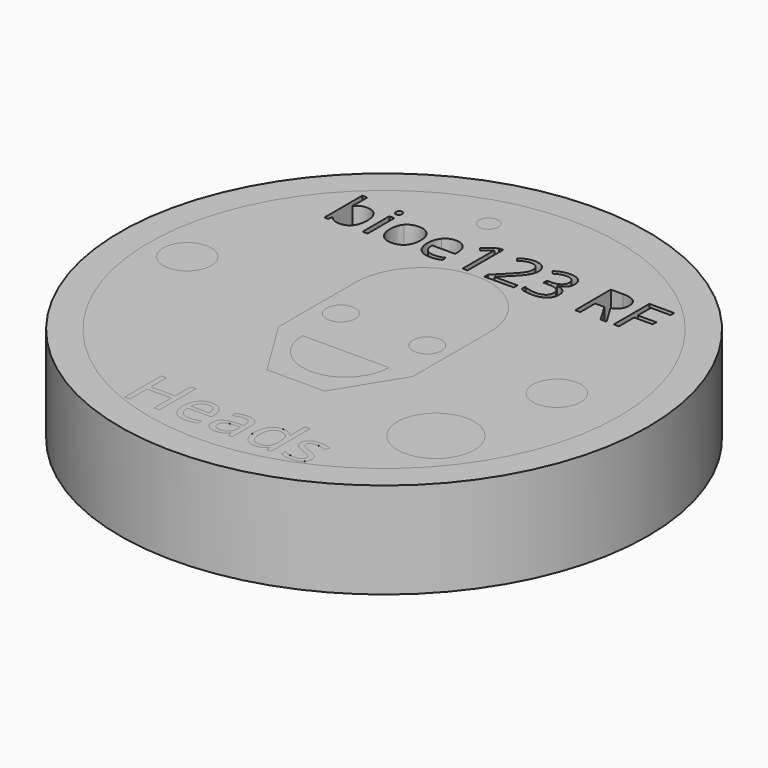
from build123d import *

# Parameters (mm, degrees)
F0_R         = 27.5
F0_R_2       = 24.5
F0_TEXT_SIZE = 6.6889777583
F0_R_3       = 4
F0_R_4       = 2.5
F0_R_5       = 1.5
F0_R_6       = 1
F1_DEPTH     = 10
F0_W         = 0.5273596823
F0_H         = 3.48016746
F2_DEPTH     = 2
F3_DEPTH     = 8


# Not quite as in the source:
# - Text() gives the source's letters only with a copy of the font that has no kerning and outlines rounded to 1/6400 em; it was checked with that copy


with BuildPart() as f1:
    # F0 (on Top) → F1 (new body)
    with BuildSketch(Plane.XY):
        Circle(F0_R)
        Circle(F0_R_2, mode=Mode.SUBTRACT)
        with Locations((-9.6953597148, -22.5)):
            Text('Heads', F0_TEXT_SIZE, font='Open Sans', text_align=(TextAlign.LEFT, TextAlign.BOTTOM))
        with Locations((15, -12)):
            Circle(F0_R_3)
        with Locations((18, 0)):
            Circle(F0_R_4)
        with BuildLine():
            Line((-3, -11.5), (3, -11.5))
            Line((3, -11.5), (7, -5))
            Line((7, -5), (7, 5))
            ThreePointArc((7, 5), (0, 12), (-7, 5))
            Line((-7, 5), (-7, -5))
            Line((-7, -5), (-3, -11.5))
        make_face()
        with BuildLine():
            Line((-4.5, -5), (4.5, -5))
            ThreePointArc((4.5, -5), (0, -9.5), (-4.5, -5))
        make_face(mode=Mode.SUBTRACT)
        with Locations((-4.5, 0)):
            Circle(F0_R_5, mode=Mode.SUBTRACT)
        with Locations((4.5, 0)):
            Circle(F0_R_5, mode=Mode.SUBTRACT)
        with Locations((-20.5, 0)):
            Circle(F0_R_4)
        with Locations((-5, 19.8808953521)):
            Circle(F0_R_6)
    extrude(amount=F1_DEPTH)

    # F0 (on Top) → F2 (join)
    with BuildSketch(Plane.XY):
        Circle(F0_R_2)
        with BuildLine():
            add(Edge.make_bspline(
                [(-2.0542477787, -22.5114966805), (-2.3103102086, -22.5658446248), (-2.6729782214, -22.5658446248)],
                knots=[0, 0, 0, 1, 1, 1], degree=2))
            add(Edge.make_bspline(
                [(-2.6729782214, -22.5658446248), (-3.4662491774, -22.5658446248), (-3.9255938219, -22.0819388901)],
                knots=[0, 0, 0, 1, 1, 1], degree=2))
            add(Edge.make_bspline(
                [(-3.9255938219, -22.0819388901), (-4.3849384664, -21.5980331554), (-4.3849384664, -20.7399627273)],
                knots=[0, 0, 0, 1, 1, 1], degree=2))
            add(Edge.make_bspline(
                [(-4.3849384664, -20.7399627273), (-4.3849384664, -19.8735310771), (-3.9585161343, -19.3640190994)],
                knots=[0, 0, 0, 1, 1, 1], degree=2))
            add(Edge.make_bspline(
                [(-3.9585161343, -19.3640190994), (-3.5320938022, -18.8545071217), (-2.8130286932, -18.8545071217)],
                knots=[0, 0, 0, 1, 1, 1], degree=2))
            add(Edge.make_bspline(
                [(-2.8130286932, -18.8545071217), (-2.140995459, -18.8545071217), (-1.7490631685, -19.2971293218)],
                knots=[0, 0, 0, 1, 1, 1], degree=2))
            add(Edge.make_bspline(
                [(-1.7490631685, -19.2971293218), (-1.357130878, -19.7397515219), (-1.357130878, -20.4650875476)],
                knots=[0, 0, 0, 1, 1, 1], degree=2))
            Line((-1.357130878, -20.4650875476), (-1.357130878, -20.8078976577))
            Line((-1.357130878, -20.8078976577), (-3.8226462736, -20.8078976577))
            add(Edge.make_bspline(
                [(-3.8226462736, -20.8078976577), (-3.8059238292, -21.4381247809), (-3.5038746773, -21.764735023)],
                knots=[0, 0, 0, 1, 1, 1], degree=2))
            add(Edge.make_bspline(
                [(-3.5038746773, -21.764735023), (-3.2018255254, -22.0913452651), (-2.6531203187, -22.0913452651)],
                knots=[0, 0, 0, 1, 1, 1], degree=2))
            add(Edge.make_bspline(
                [(-2.6531203187, -22.0913452651), (-2.0751508342, -22.0913452651), (-1.5107683359, -21.8499149741)],
                knots=[0, 0, 0, 1, 1, 1], degree=2))
            Line((-1.5107683359, -21.8499149741), (-1.5107683359, -22.3338207088))
            add(Edge.make_bspline(
                [(-1.5107683359, -22.3338207088), (-1.7981853489, -22.4571487362), (-2.0542477787, -22.5114966805)],
                knots=[0, 0, 0, 1, 1, 1], degree=2))
        make_face(mode=Mode.SUBTRACT)
        Polygon((-5.4133687967, -17.7246969722), (-5.4133687967, -22.5), (-5.9683449201, -22.5), (-5.9683449201, -20.2529215343), (-8.4840276489, -20.2529215343), (-8.4840276489, -22.5), (-9.0390037723, -22.5), (-9.0390037723, -17.7246969722), (-8.4840276489, -17.7246969722), (-8.4840276489, -19.7564739663), (-5.9683449201, -19.7564739663), (-5.9683449201, -17.7246969722), align=None, mode=Mode.SUBTRACT)
        with BuildLine():
            Line((2.1713048895, -22.5), (1.7689210712, -22.5))
            Line((1.7689210712, -22.5), (1.6612703354, -21.9899654459))
            Line((1.6612703354, -21.9899654459), (1.6351415161, -21.9899654459))
            add(Edge.make_bspline(
                [(1.6351415161, -21.9899654459), (1.3675824057, -22.3265046394), (1.1015910246, -22.4461746321)],
                knots=[0, 0, 0, 1, 1, 1], degree=2))
            add(Edge.make_bspline(
                [(1.1015910246, -22.4461746321), (0.8355996434, -22.5658446248), (0.4363512835, -22.5658446248)],
                knots=[0, 0, 0, 1, 1, 1], degree=2))
            add(Edge.make_bspline(
                [(0.4363512835, -22.5658446248), (-0.0956314789, -22.5658446248), (-0.3976806308, -22.2909694451)],
                knots=[0, 0, 0, 1, 1, 1], degree=2))
            add(Edge.make_bspline(
                [(-0.3976806308, -22.2909694451), (-0.6997297827, -22.0160942653), (-0.6997297827, -21.5102403223)],
                knots=[0, 0, 0, 1, 1, 1], degree=2))
            add(Edge.make_bspline(
                [(-0.6997297827, -21.5102403223), (-0.6997297827, -20.4264168949), (1.0341786706, -20.3741592562)],
                knots=[0, 0, 0, 1, 1, 1], degree=2))
            Line((1.0341786706, -20.3741592562), (1.6414124327, -20.3543013535))
            Line((1.6414124327, -20.3543013535), (1.6414124327, -20.1316838124))
            add(Edge.make_bspline(
                [(1.6414124327, -20.1316838124), (1.6414124327, -19.7104872442), (1.4606010027, -19.5098179115)],
                knots=[0, 0, 0, 1, 1, 1], degree=2))
            add(Edge.make_bspline(
                [(1.4606010027, -19.5098179115), (1.2797895727, -19.3091485787), (0.8805412127, -19.3091485787)],
                knots=[0, 0, 0, 1, 1, 1], degree=2))
            add(Edge.make_bspline(
                [(0.8805412127, -19.3091485787), (0.4332158251, -19.3091485787), (-0.1311666732, -19.5829786057)],
                knots=[0, 0, 0, 1, 1, 1], degree=2))
            Line((-0.1311666732, -19.5829786057), (-0.2983911172, -19.1680529541))
            add(Edge.make_bspline(
                [(-0.2983911172, -19.1680529541), (-0.0339674652, -19.024867024), (0.2811460964, -18.9433451076)],
                knots=[0, 0, 0, 1, 1, 1], degree=2))
            add(Edge.make_bspline(
                [(0.2811460964, -18.9433451076), (0.596259658, -18.8618231911), (0.9139861015, -18.8618231911)],
                knots=[0, 0, 0, 1, 1, 1], degree=2))
            add(Edge.make_bspline(
                [(0.9139861015, -18.8618231911), (1.5536195996, -18.8618231911), (1.8624622446, -19.1455821695)],
                knots=[0, 0, 0, 1, 1, 1], degree=2))
            add(Edge.make_bspline(
                [(1.8624622446, -19.1455821695), (2.1713048895, -19.4293411478), (2.1713048895, -20.0564328127)],
                knots=[0, 0, 0, 1, 1, 1], degree=2))
            Line((2.1713048895, -20.0564328127), (2.1713048895, -22.5))
        make_face(mode=Mode.SUBTRACT)
        with BuildLine():
            add(Edge.make_bspline(
                [(9.471697021, -20.9322708379), (9.6953597148, -21.1674302122), (9.6953597148, -21.5238273084)],
                knots=[0, 0, 0, 1, 1, 1], degree=2))
            add(Edge.make_bspline(
                [(9.6953597148, -21.5238273084), (9.6953597148, -22.0234103347), (9.323285327, -22.2946274798)],
                knots=[0, 0, 0, 1, 1, 1], degree=2))
            add(Edge.make_bspline(
                [(9.323285327, -22.2946274798), (8.9512109392, -22.5658446248), (8.2781325523, -22.5658446248)],
                knots=[0, 0, 0, 1, 1, 1], degree=2))
            add(Edge.make_bspline(
                [(8.2781325523, -22.5658446248), (7.5663835127, -22.5658446248), (7.1681803055, -22.3400916255)],
                knots=[0, 0, 0, 1, 1, 1], degree=2))
            Line((7.1681803055, -22.3400916255), (7.1681803055, -21.8373731408))
            add(Edge.make_bspline(
                [(7.1681803055, -21.8373731408), (7.4263330409, -21.9680172377), (7.7215886997, -22.0427456611)],
                knots=[0, 0, 0, 1, 1, 1], degree=2))
            add(Edge.make_bspline(
                [(7.7215886997, -22.0427456611), (8.0168443586, -22.1174740844), (8.2917195384, -22.1174740844)],
                knots=[0, 0, 0, 1, 1, 1], degree=2))
            add(Edge.make_bspline(
                [(8.2917195384, -22.1174740844), (8.7160515649, -22.1174740844), (8.9444174462, -21.9821268001)],
                knots=[0, 0, 0, 1, 1, 1], degree=2))
            add(Edge.make_bspline(
                [(8.9444174462, -21.9821268001), (9.1727833275, -21.8467795158), (9.1727833275, -21.5687688777)],
                knots=[0, 0, 0, 1, 1, 1], degree=2))
            add(Edge.make_bspline(
                [(9.1727833275, -21.5687688777), (9.1727833275, -21.3597383228), (8.9919718974, -21.2113266288)],
                knots=[0, 0, 0, 1, 1, 1], degree=2))
            add(Edge.make_bspline(
                [(8.9919718974, -21.2113266288), (8.8111604674, -21.0629149347), (8.2844034689, -20.8601552964)],
                knots=[0, 0, 0, 1, 1, 1], degree=2))
            add(Edge.make_bspline(
                [(8.2844034689, -20.8601552964), (7.7848204426, -20.6741181025), (7.5742221585, -20.5351127835)],
                knots=[0, 0, 0, 1, 1, 1], degree=2))
            add(Edge.make_bspline(
                [(7.5742221585, -20.5351127835), (7.3636238744, -20.3961074645), (7.2606763261, -20.2199992219)],
                knots=[0, 0, 0, 1, 1, 1], degree=2))
            add(Edge.make_bspline(
                [(7.2606763261, -20.2199992219), (7.1577287778, -20.0438909794), (7.1577287778, -19.7993252301)],
                knots=[0, 0, 0, 1, 1, 1], degree=2))
            add(Edge.make_bspline(
                [(7.1577287778, -19.7993252301), (7.1577287778, -19.3614062175), (7.514125874, -19.1079566696)],
                knots=[0, 0, 0, 1, 1, 1], degree=2))
            add(Edge.make_bspline(
                [(7.514125874, -19.1079566696), (7.8705229701, -18.8545071217), (8.4902985656, -18.8545071217)],
                knots=[0, 0, 0, 1, 1, 1], degree=2))
            add(Edge.make_bspline(
                [(8.4902985656, -18.8545071217), (9.06826805, -18.8545071217), (9.6211538678, -19.089666496)],
                knots=[0, 0, 0, 1, 1, 1], degree=2))
            Line((9.6211538678, -19.089666496), (9.4278006045, -19.530720967))
            add(Edge.make_bspline(
                [(9.4278006045, -19.530720967), (8.8895469255, -19.3091485787), (8.4516279129, -19.3091485787)],
                knots=[0, 0, 0, 1, 1, 1], degree=2))
            add(Edge.make_bspline(
                [(8.4516279129, -19.3091485787), (8.065966539, -19.3091485787), (7.8700003938, -19.4298637242)],
                knots=[0, 0, 0, 1, 1, 1], degree=2))
            add(Edge.make_bspline(
                [(7.8700003938, -19.4298637242), (7.6740342485, -19.5505788697), (7.6740342485, -19.762744883)],
                knots=[0, 0, 0, 1, 1, 1], degree=2))
            add(Edge.make_bspline(
                [(7.6740342485, -19.762744883), (7.6740342485, -19.9069759659), (7.7477175191, -20.0078332086)],
                knots=[0, 0, 0, 1, 1, 1], degree=2))
            add(Edge.make_bspline(
                [(7.7477175191, -20.0078332086), (7.8214007897, -20.1086904514), (7.9844446226, -20.2001413192)],
                knots=[0, 0, 0, 1, 1, 1], degree=2))
            add(Edge.make_bspline(
                [(7.9844446226, -20.2001413192), (8.1474884554, -20.291592187), (8.6115362874, -20.4650875476)],
                knots=[0, 0, 0, 1, 1, 1], degree=2))
            add(Edge.make_bspline(
                [(8.6115362874, -20.4650875476), (9.2480343272, -20.6971114636), (9.471697021, -20.9322708379)],
                knots=[0, 0, 0, 1, 1, 1], degree=2))
        make_face(mode=Mode.SUBTRACT)
        with BuildLine():
            Line((5.7958947123, -22.5), (5.7237791708, -22.0202748764))
            Line((5.7237791708, -22.0202748764), (5.6945148931, -22.0202748764))
            add(Edge.make_bspline(
                [(5.6945148931, -22.0202748764), (5.319305047, -22.5658446248), (4.5709756603, -22.5658446248)],
                knots=[0, 0, 0, 1, 1, 1], degree=2))
            add(Edge.make_bspline(
                [(4.5709756603, -22.5658446248), (3.8686329957, -22.5658446248), (3.4782684343, -22.0855969248)],
                knots=[0, 0, 0, 1, 1, 1], degree=2))
            add(Edge.make_bspline(
                [(3.4782684343, -22.0855969248), (3.087903873, -21.6053492248), (3.087903873, -20.7201048246)],
                knots=[0, 0, 0, 1, 1, 1], degree=2))
            add(Edge.make_bspline(
                [(3.087903873, -20.7201048246), (3.087903873, -19.8348604244), (3.4798361635, -19.3446837731)],
                knots=[0, 0, 0, 1, 1, 1], degree=2))
            add(Edge.make_bspline(
                [(3.4798361635, -19.3446837731), (3.871768454, -18.8545071217), (4.5709756603, -18.8545071217)],
                knots=[0, 0, 0, 1, 1, 1], degree=2))
            add(Edge.make_bspline(
                [(4.5709756603, -18.8545071217), (5.2994471443, -18.8545071217), (5.6882439765, -19.3843995785)],
                knots=[0, 0, 0, 1, 1, 1], degree=2))
            Line((5.6882439765, -19.3843995785), (5.7310952403, -19.3843995785))
            Line((5.7310952403, -19.3843995785), (5.7081018792, -19.1262468432))
            Line((5.7081018792, -19.1262468432), (5.6945148931, -18.8743650244))
            Line((5.6945148931, -18.8743650244), (5.6945148931, -17.4174220565))
            Line((5.6945148931, -17.4174220565), (6.2369491832, -17.4174220565))
            Line((6.2369491832, -17.4174220565), (6.2369491832, -22.5))
            Line((6.2369491832, -22.5), (5.7958947123, -22.5))
        make_face(mode=Mode.SUBTRACT)
        with Locations((15, -12)):
            Circle(F0_R_3, mode=Mode.SUBTRACT)
        with Locations((-20.5, 0)):
            Circle(F0_R_4, mode=Mode.SUBTRACT)
        with BuildLine():
            add(Edge.make_bspline(
                [(-15.5855990593, 15.3794973469), (-15.2177682212, 15.8997442781), (-14.4932837251, 15.8997442781)],
                knots=[0, 0, 0, 1, 1, 1], degree=2))
            add(Edge.make_bspline(
                [(-14.4932837251, 15.8997442781), (-13.807411306, 15.8997442781), (-13.4278952341, 15.4313188185)],
                knots=[0, 0, 0, 1, 1, 1], degree=2))
            add(Edge.make_bspline(
                [(-13.4278952341, 15.4313188185), (-13.0483791622, 14.9628933589), (-13.0483791622, 14.1063149155)],
                knots=[0, 0, 0, 1, 1, 1], degree=2))
            add(Edge.make_bspline(
                [(-13.0483791622, 14.1063149155), (-13.0483791622, 13.2487203648), (-13.430943556, 12.7736902078)],
                knots=[0, 0, 0, 1, 1, 1], degree=2))
            add(Edge.make_bspline(
                [(-13.430943556, 12.7736902078), (-13.8135079497, 12.2986600509), (-14.4932837251, 12.2986600509)],
                knots=[0, 0, 0, 1, 1, 1], degree=2))
            add(Edge.make_bspline(
                [(-14.4932837251, 12.2986600509), (-14.8336796665, 12.2986600509), (-15.1146333315, 12.4241493009)],
                knots=[0, 0, 0, 1, 1, 1], degree=2))
            add(Edge.make_bspline(
                [(-15.1146333315, 12.4241493009), (-15.3955869965, 12.5496385509), (-15.5855990593, 12.8107781238)],
                knots=[0, 0, 0, 1, 1, 1], degree=2))
            Line((-15.5855990593, 12.8107781238), (-15.6242111362, 12.8107781238))
            Line((-15.6242111362, 12.8107781238), (-15.7349668306, 12.36267481))
            Line((-15.7349668306, 12.36267481), (-16.1129587416, 12.36267481))
            Line((-16.1129587416, 12.36267481), (-16.1129587416, 17.3040045496))
            Line((-16.1129587416, 17.3040045496), (-15.5855990593, 17.3040045496))
            Line((-15.5855990593, 17.3040045496), (-15.5855990593, 16.1029657356))
            add(Edge.make_bspline(
                [(-15.5855990593, 16.1029657356), (-15.5855990593, 15.6995711425), (-15.6110017415, 15.3794973469)],
                knots=[0, 0, 0, 1, 1, 1], degree=2))
            Line((-15.6110017415, 15.3794973469), (-15.5855990593, 15.3794973469))
        make_face(mode=Mode.SUBTRACT)
        with Locations((-11.8641061185, 14.10275854)):
            Rectangle(F0_W, F0_H, mode=Mode.SUBTRACT)
        with BuildLine():
            add(Edge.make_bspline(
                [(-12.0835852926, 16.5205858308), (-12.1724946803, 16.6079710576), (-12.1724946803, 16.7857898329)],
                knots=[0, 0, 0, 1, 1, 1], degree=2))
            add(Edge.make_bspline(
                [(-12.1724946803, 16.7857898329), (-12.1724946803, 16.9666569301), (-12.0835852926, 17.050993835)],
                knots=[0, 0, 0, 1, 1, 1], degree=2))
            add(Edge.make_bspline(
                [(-12.0835852926, 17.050993835), (-11.9946759049, 17.1353307398), (-11.860549743, 17.1353307398)],
                knots=[0, 0, 0, 1, 1, 1], degree=2))
            add(Edge.make_bspline(
                [(-11.860549743, 17.1353307398), (-11.733536332, 17.1353307398), (-11.6415786225, 17.049469674)],
                knots=[0, 0, 0, 1, 1, 1], degree=2))
            add(Edge.make_bspline(
                [(-11.6415786225, 17.049469674), (-11.549620913, 16.9636086082), (-11.549620913, 16.7857898329)],
                knots=[0, 0, 0, 1, 1, 1], degree=2))
            add(Edge.make_bspline(
                [(-11.549620913, 16.7857898329), (-11.549620913, 16.6079710576), (-11.6415786225, 16.5205858308)],
                knots=[0, 0, 0, 1, 1, 1], degree=2))
            add(Edge.make_bspline(
                [(-11.6415786225, 16.5205858308), (-11.733536332, 16.4332006041), (-11.860549743, 16.4332006041)],
                knots=[0, 0, 0, 1, 1, 1], degree=2))
            add(Edge.make_bspline(
                [(-11.860549743, 16.4332006041), (-11.9946759049, 16.4332006041), (-12.0835852926, 16.5205858308)],
                knots=[0, 0, 0, 1, 1, 1], degree=2))
        make_face(mode=Mode.SUBTRACT)
        with BuildLine():
            add(Edge.make_bspline(
                [(-7.9094165552, 15.420649692), (-7.4790951189, 14.9344423549), (-7.4790951189, 14.1063149155)],
                knots=[0, 0, 0, 1, 1, 1], degree=2))
            add(Edge.make_bspline(
                [(-7.4790951189, 14.1063149155), (-7.4790951189, 13.2548170085), (-7.9073843406, 12.7767385297)],
                knots=[0, 0, 0, 1, 1, 1], degree=2))
            add(Edge.make_bspline(
                [(-7.9073843406, 12.7767385297), (-8.3356735623, 12.2986600509), (-9.0916573843, 12.2986600509)],
                knots=[0, 0, 0, 1, 1, 1], degree=2))
            add(Edge.make_bspline(
                [(-9.0916573843, 12.2986600509), (-9.5590667366, 12.2986600509), (-9.920800931, 12.518139225)],
                knots=[0, 0, 0, 1, 1, 1], degree=2))
            add(Edge.make_bspline(
                [(-9.920800931, 12.518139225), (-10.2825351253, 12.7376183991), (-10.4796599391, 13.147109636)],
                knots=[0, 0, 0, 1, 1, 1], degree=2))
            add(Edge.make_bspline(
                [(-10.4796599391, 13.147109636), (-10.6767847529, 13.5566008729), (-10.6767847529, 14.1063149155)],
                knots=[0, 0, 0, 1, 1, 1], degree=2))
            add(Edge.make_bspline(
                [(-10.6767847529, 14.1063149155), (-10.6767847529, 14.9567967152), (-10.2510357994, 15.4318268722)],
                knots=[0, 0, 0, 1, 1, 1], degree=2))
            add(Edge.make_bspline(
                [(-10.2510357994, 15.4318268722), (-9.8252868459, 15.9068570291), (-9.069303024, 15.9068570291)],
                knots=[0, 0, 0, 1, 1, 1], degree=2))
            add(Edge.make_bspline(
                [(-9.069303024, 15.9068570291), (-8.3397379915, 15.9068570291), (-7.9094165552, 15.420649692)],
                knots=[0, 0, 0, 1, 1, 1], degree=2))
        make_face(mode=Mode.SUBTRACT)
        with BuildLine():
            add(Edge.make_bspline(
                [(-4.4825947278, 12.3514976298), (-4.7315410132, 12.2986600509), (-5.084130242, 12.2986600509)],
                knots=[0, 0, 0, 1, 1, 1], degree=2))
            add(Edge.make_bspline(
                [(-5.084130242, 12.2986600509), (-5.8553556733, 12.2986600509), (-6.3019348262, 12.769117725)],
                knots=[0, 0, 0, 1, 1, 1], degree=2))
            add(Edge.make_bspline(
                [(-6.3019348262, 12.769117725), (-6.7485139791, 13.2395753992), (-6.7485139791, 14.0737994823)],
                knots=[0, 0, 0, 1, 1, 1], degree=2))
            add(Edge.make_bspline(
                [(-6.7485139791, 14.0737994823), (-6.7485139791, 14.9161524237), (-6.3339422058, 15.4115047264)],
                knots=[0, 0, 0, 1, 1, 1], degree=2))
            add(Edge.make_bspline(
                [(-6.3339422058, 15.4115047264), (-5.9193704324, 15.9068570291), (-5.2202886186, 15.9068570291)],
                knots=[0, 0, 0, 1, 1, 1], degree=2))
            add(Edge.make_bspline(
                [(-5.2202886186, 15.9068570291), (-4.5669316326, 15.9068570291), (-4.1858913998, 15.4765355928)],
                knots=[0, 0, 0, 1, 1, 1], degree=2))
            add(Edge.make_bspline(
                [(-4.1858913998, 15.4765355928), (-3.8048511669, 15.0462141565), (-3.8048511669, 14.3410356989)],
                knots=[0, 0, 0, 1, 1, 1], degree=2))
            Line((-3.8048511669, 14.3410356989), (-3.8048511669, 14.0077525086))
            Line((-3.8048511669, 14.0077525086), (-6.2018482584, 14.0077525086))
            add(Edge.make_bspline(
                [(-6.2018482584, 14.0077525086), (-6.1855905418, 13.3950398142), (-5.8919355357, 13.0775062868)],
                knots=[0, 0, 0, 1, 1, 1], degree=2))
            add(Edge.make_bspline(
                [(-5.8919355357, 13.0775062868), (-5.5982805295, 12.7599727594), (-5.0648242035, 12.7599727594)],
                knots=[0, 0, 0, 1, 1, 1], degree=2))
            add(Edge.make_bspline(
                [(-5.0648242035, 12.7599727594), (-4.5029168735, 12.7599727594), (-3.9542189382, 12.9946935429)],
                knots=[0, 0, 0, 1, 1, 1], degree=2))
            Line((-3.9542189382, 12.9946935429), (-3.9542189382, 12.5242358687))
            add(Edge.make_bspline(
                [(-3.9542189382, 12.5242358687), (-4.2336484423, 12.4043352088), (-4.4825947278, 12.3514976298)],
                knots=[0, 0, 0, 1, 1, 1], degree=2))
        make_face(mode=Mode.SUBTRACT)
        with BuildLine():
            Line((-1.1944715451, 17.005269007), (-1.1944715451, 12.36267481))
            Line((-1.1944715451, 12.36267481), (-1.7086218326, 12.36267481))
            Line((-1.7086218326, 12.36267481), (-1.7086218326, 15.6711201384))
            add(Edge.make_bspline(
                [(-1.7086218326, 15.6711201384), (-1.7086218326, 16.0846758044), (-1.6832191504, 16.4525066426)],
                knots=[0, 0, 0, 1, 1, 1], degree=2))
            add(Edge.make_bspline(
                [(-1.6832191504, 16.4525066426), (-1.7492661241, 16.3854435616), (-1.8320788681, 16.3127918905)],
                knots=[0, 0, 0, 1, 1, 1], degree=2))
            add(Edge.make_bspline(
                [(-1.8320788681, 16.3127918905), (-1.914891612, 16.2401402195), (-2.5875546364, 15.6934744987)],
                knots=[0, 0, 0, 1, 1, 1], degree=2))
            Line((-2.5875546364, 15.6934744987), (-2.8669841405, 16.0552086931))
            Line((-2.8669841405, 16.0552086931), (-1.6385104298, 17.005269007))
            Line((-1.6385104298, 17.005269007), (-1.1944715451, 17.005269007))
        make_face(mode=Mode.SUBTRACT)
        with Locations((-5, 19.8808953521)):
            Circle(F0_R_6, mode=Mode.SUBTRACT)
        with BuildLine():
            Line((7, -5), (3, -11.5))
            Line((3, -11.5), (-3, -11.5))
            Line((-3, -11.5), (-7, -5))
            Line((-7, -5), (-7, 5))
            ThreePointArc((-7, 5), (0, 12), (7, 5))
            Line((7, 5), (7, -5))
        make_face(mode=Mode.SUBTRACT)
        with Locations((18, 0)):
            Circle(F0_R_4, mode=Mode.SUBTRACT)
        with BuildLine():
            Line((3.6228931054, 12.8514224153), (3.6228931054, 12.36267481))
            Line((3.6228931054, 12.36267481), (0.5715229207, 12.36267481))
            Line((0.5715229207, 12.36267481), (0.5715229207, 12.8168747675))
            Line((0.5715229207, 12.8168747675), (1.7938999877, 14.0453484782))
            add(Edge.make_bspline(
                [(1.7938999877, 14.0453484782), (2.3527589959, 14.6113202374), (2.5305777712, 14.8526457182)],
                knots=[0, 0, 0, 1, 1, 1], degree=2))
            add(Edge.make_bspline(
                [(2.5305777712, 14.8526457182), (2.7083965465, 15.093971199), (2.7973059342, 15.3225953388)],
                knots=[0, 0, 0, 1, 1, 1], degree=2))
            add(Edge.make_bspline(
                [(2.7973059342, 15.3225953388), (2.8862153219, 15.5512194785), (2.8862153219, 15.8143912659)],
                knots=[0, 0, 0, 1, 1, 1], degree=2))
            add(Edge.make_bspline(
                [(2.8862153219, 15.8143912659), (2.8862153219, 16.1862865332), (2.660639504, 16.4037334928)],
                knots=[0, 0, 0, 1, 1, 1], degree=2))
            add(Edge.make_bspline(
                [(2.660639504, 16.4037334928), (2.4350636862, 16.6211804523), (2.0347174149, 16.6211804523)],
                knots=[0, 0, 0, 1, 1, 1], degree=2))
            add(Edge.make_bspline(
                [(2.0347174149, 16.6211804523), (1.7461429452, 16.6211804523), (1.4870355869, 16.5256663673)],
                knots=[0, 0, 0, 1, 1, 1], degree=2))
            add(Edge.make_bspline(
                [(1.4870355869, 16.5256663673), (1.2279282285, 16.4301522822), (0.9109027548, 16.1791737822)],
                knots=[0, 0, 0, 1, 1, 1], degree=2))
            Line((0.9109027548, 16.1791737822), (0.6314732507, 16.5378596547))
            add(Edge.make_bspline(
                [(0.6314732507, 16.5378596547), (1.2726369492, 17.0713159807), (2.0286207711, 17.0713159807)],
                knots=[0, 0, 0, 1, 1, 1], degree=2))
            add(Edge.make_bspline(
                [(2.0286207711, 17.0713159807), (2.6829938644, 17.0713159807), (3.054381078, 16.7365086294)],
                knots=[0, 0, 0, 1, 1, 1], degree=2))
            add(Edge.make_bspline(
                [(3.054381078, 16.7365086294), (3.4257682916, 16.4017012782), (3.4257682916, 15.8367456263)],
                knots=[0, 0, 0, 1, 1, 1], degree=2))
            add(Edge.make_bspline(
                [(3.4257682916, 15.8367456263), (3.4257682916, 15.3947389562), (3.1778381134, 14.9628933589)],
                knots=[0, 0, 0, 1, 1, 1], degree=2))
            add(Edge.make_bspline(
                [(3.1778381134, 14.9628933589), (2.9299079352, 14.5310477617), (2.2511482671, 13.8705780248)],
                knots=[0, 0, 0, 1, 1, 1], degree=2))
            Line((2.2511482671, 13.8705780248), (1.2350409795, 12.8768250975))
            Line((1.2350409795, 12.8768250975), (1.2350409795, 12.8514224153))
            Line((1.2350409795, 12.8514224153), (3.6228931054, 12.8514224153))
        make_face(mode=Mode.SUBTRACT)
        with BuildLine():
            add(Edge.make_bspline(
                [(6.7911156281, 16.7619113116), (7.1660592172, 16.4525066426), (7.1660592172, 15.9129536728)],
                knots=[0, 0, 0, 1, 1, 1], degree=2))
            add(Edge.make_bspline(
                [(7.1660592172, 15.9129536728), (7.1660592172, 15.4678986809), (6.9166048781, 15.1854208549)],
                knots=[0, 0, 0, 1, 1, 1], degree=2))
            add(Edge.make_bspline(
                [(6.9166048781, 15.1854208549), (6.667150539, 14.902943029), (6.2099022596, 14.8074289439)],
                knots=[0, 0, 0, 1, 1, 1], degree=2))
            Line((6.2099022596, 14.8074289439), (6.2099022596, 14.7820262618))
            add(Edge.make_bspline(
                [(6.2099022596, 14.7820262618), (6.7687612678, 14.7129309662), (7.0385377526, 14.4268967647)],
                knots=[0, 0, 0, 1, 1, 1], degree=2))
            add(Edge.make_bspline(
                [(7.0385377526, 14.4268967647), (7.3083142375, 14.1408625633), (7.3083142375, 13.6775176401)],
                knots=[0, 0, 0, 1, 1, 1], degree=2))
            add(Edge.make_bspline(
                [(7.3083142375, 13.6775176401), (7.3083142375, 13.0139995813), (6.8480176362, 12.6563298161)],
                knots=[0, 0, 0, 1, 1, 1], degree=2))
            add(Edge.make_bspline(
                [(6.8480176362, 12.6563298161), (6.3877210349, 12.2986600509), (5.5402875571, 12.2986600509)],
                knots=[0, 0, 0, 1, 1, 1], degree=2))
            add(Edge.make_bspline(
                [(5.5402875571, 12.2986600509), (5.1714406117, 12.2986600509), (4.8650842645, 12.3545459517)],
                knots=[0, 0, 0, 1, 1, 1], degree=2))
            add(Edge.make_bspline(
                [(4.8650842645, 12.3545459517), (4.5587279173, 12.4104318525), (4.2701534476, 12.5496385509)],
                knots=[0, 0, 0, 1, 1, 1], degree=2))
            Line((4.2701534476, 12.5496385509), (4.2701534476, 13.051595551))
            add(Edge.make_bspline(
                [(4.2701534476, 13.051595551), (4.571937312, 12.9022277797), (4.9133493606, 12.8244955722)],
                knots=[0, 0, 0, 1, 1, 1], degree=2))
            add(Edge.make_bspline(
                [(4.9133493606, 12.8244955722), (5.2547614093, 12.7467633647), (5.5595935955, 12.7467633647)],
                knots=[0, 0, 0, 1, 1, 1], degree=2))
            add(Edge.make_bspline(
                [(5.5595935955, 12.7467633647), (6.762664624, 12.7467633647), (6.762664624, 13.6897109276)],
                knots=[0, 0, 0, 1, 1, 1], degree=2))
            add(Edge.make_bspline(
                [(6.762664624, 13.6897109276), (6.762664624, 14.5351121909), (5.4356285064, 14.5351121909)],
                knots=[0, 0, 0, 1, 1, 1], degree=2))
            Line((5.4356285064, 14.5351121909), (4.978380227, 14.5351121909))
            Line((4.978380227, 14.5351121909), (4.978380227, 14.9882960411))
            Line((4.978380227, 14.9882960411), (5.4417251502, 14.9882960411))
            add(Edge.make_bspline(
                [(5.4417251502, 14.9882960411), (5.9843264417, 14.9882960411), (6.3018599691, 15.228097361)],
                knots=[0, 0, 0, 1, 1, 1], degree=2))
            add(Edge.make_bspline(
                [(6.3018599691, 15.228097361), (6.6193934965, 15.4678986809), (6.6193934965, 15.8936476344)],
                knots=[0, 0, 0, 1, 1, 1], degree=2))
            add(Edge.make_bspline(
                [(6.6193934965, 15.8936476344), (6.6193934965, 16.2330274684), (6.386196874, 16.4271039604)],
                knots=[0, 0, 0, 1, 1, 1], degree=2))
            add(Edge.make_bspline(
                [(6.386196874, 16.4271039604), (6.1530002515, 16.6211804523), (5.7526539802, 16.6211804523)],
                knots=[0, 0, 0, 1, 1, 1], degree=2))
            add(Edge.make_bspline(
                [(5.7526539802, 16.6211804523), (5.4478217939, 16.6211804523), (5.178045309, 16.5383677084)],
                knots=[0, 0, 0, 1, 1, 1], degree=2))
            add(Edge.make_bspline(
                [(5.178045309, 16.5383677084), (4.9082688242, 16.4555549644), (4.5617762391, 16.2330274684)],
                knots=[0, 0, 0, 1, 1, 1], degree=2))
            Line((4.5617762391, 16.2330274684), (4.2955561298, 16.5886650191))
            add(Edge.make_bspline(
                [(4.2955561298, 16.5886650191), (4.5810822776, 16.8142408369), (4.9539936521, 16.9427784088)],
                knots=[0, 0, 0, 1, 1, 1], degree=2))
            add(Edge.make_bspline(
                [(4.9539936521, 16.9427784088), (5.3269050267, 17.0713159807), (5.7404606927, 17.0713159807)],
                knots=[0, 0, 0, 1, 1, 1], degree=2))
            add(Edge.make_bspline(
                [(5.7404606927, 17.0713159807), (6.416172039, 17.0713159807), (6.7911156281, 16.7619113116)],
                knots=[0, 0, 0, 1, 1, 1], degree=2))
        make_face(mode=Mode.SUBTRACT)
        with BuildLine():
            Line((11.5261755883, 14.2932786564), (10.5568092359, 14.2932786564))
            Line((10.5568092359, 14.2932786564), (10.5568092359, 12.36267481))
            Line((10.5568092359, 12.36267481), (10.0172562662, 12.36267481))
            Line((10.0172562662, 12.36267481), (10.0172562662, 17.005269007))
            Line((10.0172562662, 17.005269007), (11.2904386976, 17.005269007))
            add(Edge.make_bspline(
                [(11.2904386976, 17.005269007), (12.1449849264, 17.005269007), (12.5529520024, 16.6780824604)],
                knots=[0, 0, 0, 1, 1, 1], degree=2))
            add(Edge.make_bspline(
                [(12.5529520024, 16.6780824604), (12.9609190784, 16.3508959138), (12.9609190784, 15.6934744987)],
                knots=[0, 0, 0, 1, 1, 1], degree=2))
            add(Edge.make_bspline(
                [(12.9609190784, 15.6934744987), (12.9609190784, 14.7728812962), (12.0271164811, 14.4487430714)],
                knots=[0, 0, 0, 1, 1, 1], degree=2))
            Line((12.0271164811, 14.4487430714), (13.288105625, 12.36267481))
            Line((13.288105625, 12.36267481), (12.6499902484, 12.36267481))
            Line((12.6499902484, 12.36267481), (11.5261755883, 14.2932786564))
        make_face(mode=Mode.SUBTRACT)
        Polygon((14.5765296656, 14.3471323427), (14.5765296656, 12.36267481), (14.0369766959, 12.36267481), (14.0369766959, 17.005269007), (16.6250019574, 17.005269007), (16.6250019574, 16.5256663673), (14.5765296656, 16.5256663673), (14.5765296656, 14.8267349824), (16.5010368683, 14.8267349824), (16.5010368683, 14.3471323427), align=None, mode=Mode.SUBTRACT)
        with BuildLine():
            ThreePointArc((-4.5, -5), (0, -9.5), (4.5, -5))
            Line((4.5, -5), (-4.5, -5))
        make_face()
        with Locations((-4.5, 0)):
            Circle(F0_R_5)
        with Locations((4.5, 0)):
            Circle(F0_R_5)
        with BuildLine():
            add(Edge.make_bspline(
                [(-2.166601702, -19.5819334529), (-2.3949675833, -19.3091485787), (-2.8203447626, -19.3091485787)],
                knots=[0, 0, 0, 1, 1, 1], degree=2))
            add(Edge.make_bspline(
                [(-2.8203447626, -19.3091485787), (-3.2509477058, -19.3091485787), (-3.507532712, -19.5897720987)],
                knots=[0, 0, 0, 1, 1, 1], degree=2))
            add(Edge.make_bspline(
                [(-3.507532712, -19.5897720987), (-3.7641177182, -19.8703956188), (-3.8101044403, -20.3668431868)],
                knots=[0, 0, 0, 1, 1, 1], degree=2))
            Line((-3.8101044403, -20.3668431868), (-1.9382358207, -20.3668431868))
            add(Edge.make_bspline(
                [(-1.9382358207, -20.3668431868), (-1.9382358207, -19.8547183271), (-2.166601702, -19.5819334529)],
                knots=[0, 0, 0, 1, 1, 1], degree=2))
        make_face()
        with BuildLine():
            add(Edge.make_bspline(
                [(0.0465092985, -21.9643592029), (0.2241852702, -22.1174740844), (0.5440020192, -22.1174740844)],
                knots=[0, 0, 0, 1, 1, 1], degree=2))
            add(Edge.make_bspline(
                [(0.5440020192, -22.1174740844), (1.050901115, -22.1174740844), (1.3398858572, -21.8399860228)],
                knots=[0, 0, 0, 1, 1, 1], degree=2))
            add(Edge.make_bspline(
                [(1.3398858572, -21.8399860228), (1.6288705994, -21.5624979611), (1.6288705994, -21.0629149347)],
                knots=[0, 0, 0, 1, 1, 1], degree=2))
            Line((1.6288705994, -21.0629149347), (1.6288705994, -20.7399627273))
            Line((1.6288705994, -20.7399627273), (1.0864363093, -20.7619109356))
            add(Edge.make_bspline(
                [(1.0864363093, -20.7619109356), (0.4394867418, -20.7849042967), (0.1541600343, -20.9631028448)],
                knots=[0, 0, 0, 1, 1, 1], degree=2))
            add(Edge.make_bspline(
                [(0.1541600343, -20.9631028448), (-0.1311666732, -21.1413013928), (-0.1311666732, -21.516511239)],
                knots=[0, 0, 0, 1, 1, 1], degree=2))
            add(Edge.make_bspline(
                [(-0.1311666732, -21.516511239), (-0.1311666732, -21.8112443214), (0.0465092985, -21.9643592029)],
                knots=[0, 0, 0, 1, 1, 1], degree=2))
        make_face()
        with BuildLine():
            add(Edge.make_bspline(
                [(3.9015553081, -21.7615995646), (4.1529145504, -22.1112031678), (4.6399557434, -22.1112031678)],
                knots=[0, 0, 0, 1, 1, 1], degree=2))
            add(Edge.make_bspline(
                [(4.6399557434, -22.1112031678), (5.1949318668, -22.1112031678), (5.44472338, -21.8091540159)],
                knots=[0, 0, 0, 1, 1, 1], degree=2))
            add(Edge.make_bspline(
                [(5.44472338, -21.8091540159), (5.6945148931, -21.507104864), (5.6945148931, -20.8340264771)],
                knots=[0, 0, 0, 1, 1, 1], degree=2))
            Line((5.6945148931, -20.8340264771), (5.6945148931, -20.7201048246))
            add(Edge.make_bspline(
                [(5.6945148931, -20.7201048246), (5.6945148931, -19.9592336046), (5.4415879217, -19.6341910917)],
                knots=[0, 0, 0, 1, 1, 1], degree=2))
            add(Edge.make_bspline(
                [(5.4415879217, -19.6341910917), (5.1886609502, -19.3091485787), (4.6336848268, -19.3091485787)],
                knots=[0, 0, 0, 1, 1, 1], degree=2))
            add(Edge.make_bspline(
                [(4.6336848268, -19.3091485787), (4.1560500087, -19.3091485787), (3.9031230372, -19.6796552374)],
                knots=[0, 0, 0, 1, 1, 1], degree=2))
            add(Edge.make_bspline(
                [(3.9031230372, -19.6796552374), (3.6501960658, -20.050161896), (3.6501960658, -20.7263757413)],
                knots=[0, 0, 0, 1, 1, 1], degree=2))
            add(Edge.make_bspline(
                [(3.6501960658, -20.7263757413), (3.6501960658, -21.4119959615), (3.9015553081, -21.7615995646)],
                knots=[0, 0, 0, 1, 1, 1], degree=2))
        make_face()
    extrude(amount=F2_DEPTH)


with BuildPart() as f3:
    # F3 (new): a face of the model
    f3_faces = [f1.part.faces().sort_by_distance(p)[0] for p in [
        (-23.8070353516, 0, 2),
    ]]
    extrude(f3_faces, amount=F3_DEPTH)


with BuildPart() as f3b:
    # F3#2 (new): a face of the model
    f3_2_faces = [f1.part.faces().sort_by_distance(p)[0] for p in [
        (-4.5, 0, 2),
    ]]
    extrude(f3_2_faces, amount=F3_DEPTH)


with BuildPart() as f3c:
    # F3#3 (new): a face of the model
    f3_3_faces = [f1.part.faces().sort_by_distance(p)[0] for p in [
        (4.5, 0, 2),
    ]]
    extrude(f3_3_faces, amount=F3_DEPTH)


with BuildPart() as f3d:
    # F3#4 (new): a face of the model
    f3_4_faces = [f1.part.faces().sort_by_distance(p)[0] for p in [
        (0, -6.9098593171, 2),
    ]]
    extrude(f3_4_faces, amount=F3_DEPTH)


with BuildPart() as f3e:
    # F3#5 (new): a face of the model
    f3_5_faces = [f1.part.faces().sort_by_distance(p)[0] for p in [
        (-2.8509055733, -19.9085691178, 2),
    ]]
    extrude(f3_5_faces, amount=F3_DEPTH)


with BuildPart() as f3f:
    # F3#6 (new): a face of the model
    f3_6_faces = [f1.part.faces().sort_by_distance(p)[0] for p in [
        (0.7583874812, -21.4114499713, 2),
    ]]
    extrude(f3_6_faces, amount=F3_DEPTH)


with BuildPart() as f3g:
    # F3#7 (new): a face of the model
    f3_7_faces = [f1.part.faces().sort_by_distance(p)[0] for p in [
        (4.6801746212, -20.7162263881, 2),
    ]]
    extrude(f3_7_faces, amount=F3_DEPTH)


solid = Compound([f1.part, f3.part, f3b.part, f3c.part, f3d.part, f3e.part, f3f.part, f3g.part])
